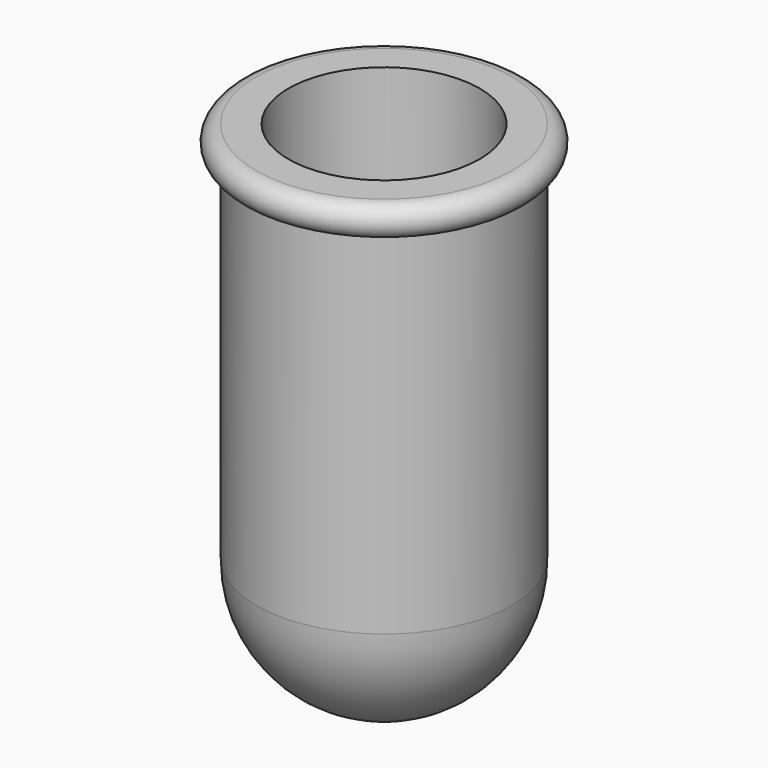
from build123d import *

# Parameters (mm, degrees)
F2_R = 12.7
F3_T = 3.175


# Not quite as in the source:
# - a shell that OpenCascade refuses in one call is made with other operations: the cavity is built on its own and cut out


with BuildPart() as f1:
    # F0 (on Front) → F1 (revolve)
    with BuildSketch(Plane.XZ):
        Polygon((0, 50.8), (0, 0), (12.7, 0), (12.7, 47.6801507175), (12.7, 50.8), align=None)
        with BuildLine():
            ThreePointArc((12.7, 47.6801507175), (14.2599246413, 49.2400753587), (12.7, 50.8))
            Line((12.7, 50.8), (12.7, 47.6801507175))
        make_face()
    revolve(axis=Axis((0, 0, 25.4), (0, 0, 1)))

    # F2
    f2_edges = [f1.edges().sort_by_distance(p)[0] for p in [
        (-12.7, 0, 0),
    ]]
    fillet(f2_edges, radius=F2_R)

    # F3: shell of thickness 3.175, made by hand


with BuildPart() as f3_core1:
    # F3_t2: copy of F1
    add(f1.part)

    # the walls: a layer under each face that stays
    f3_faces = [f3_core1.faces().sort_by_distance(p)[0] for p in [
        (-12.7, 0, 30.1900753587),
        (-8.9802561211, 0, 3.7197438789),
    ]]
    thicken(f3_faces, amount=-F3_T, mode=Mode.SUBTRACT)

    # F3_s3 → F3_t4 (revolve, cut)
    with BuildSketch(Plane.XZ):
        Polygon((12.73175, 47.6484007175), (9.525, 47.6801507175), (9.525, 50.8551507175), (12.7, 50.8551507175), align=None)
    revolve(axis=Axis((0, 0, 47.6801507175), (0, 0, 1)), mode=Mode.SUBTRACT)


with BuildPart() as f1_1:
    add(f1.part)

    # what is left inside the walls is the cavity
    f3_cavity = [f3_core1.part.solids().sort_by_distance(p)[0] for p in [
        (-9.49325, 0, 25.4),
    ]]
    add(f3_cavity, mode=Mode.SUBTRACT)


solid = f1_1.part
